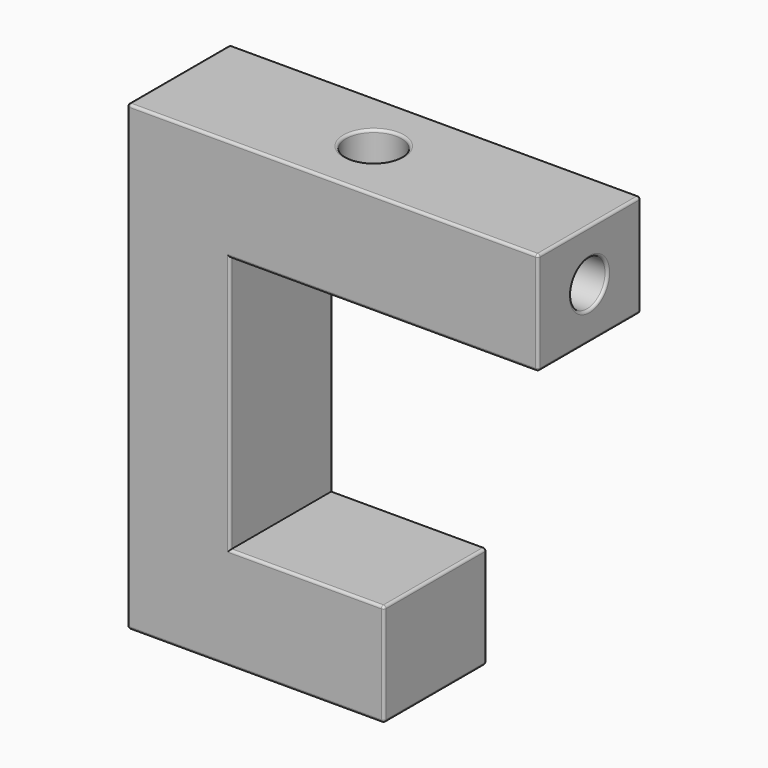
from build123d import *

# Parameters (mm, degrees)
F1_DEPTH = 25
F3_D     = 10.8
F3_DEPTH = 21
F3_TIP   = 3.2446473427
F5_D     = 8.8
F5_DEPTH = 21
F5_TIP   = 2.6437867237
F6_R     = 0.5


with BuildPart() as f1:
    # F0 (on Front) → F1 (new body)
    with BuildSketch(Plane.XZ):
        Polygon((0, -20), (0, 0), (-30, 0), (-30, 50), (30, 50), (30, 70), (-50, 70), (-50, -20), align=None)
    extrude(amount=F1_DEPTH)

    # F3 (one way)
    with BuildSketch(Plane(origin=(0, 0, 50), x_dir=(1, 0, 0), z_dir=(0, 0, -1))):
        with Locations((-12, 12.5)):
            Circle(F3_D / 2)
    extrude(amount=-F3_DEPTH, mode=Mode.SUBTRACT)
    with Locations(Plane(origin=(0, 0, 50), x_dir=(1, 0, 0), z_dir=(0, 0, -1))):
        with Locations((-12, 12.5)):
            with Locations((0, 0, -(F3_DEPTH + F3_TIP / 2))):  # 118° drill point
                Cone(0, F3_D / 2, F3_TIP, mode=Mode.SUBTRACT)

    # F5
    with Locations(Plane.YZ.offset(30)):
        with Locations((-12.5, 60)):
            Hole(F5_D / 2, depth=F5_DEPTH)
            with Locations((0, 0, -(F5_DEPTH + F5_TIP / 2))):  # 118° drill point
                Cone(0, F5_D / 2, F5_TIP, mode=Mode.SUBTRACT)

    # F6
    f6_edges = [f1.edges().sort_by_distance(p)[0] for p in [
        (0, -25, -10),
        (-15, -25, 0),
        (-30, -25, 25),
        (0, -25, 50),
        (30, -25, 60),
        (-10, -25, 70),
        (-50, -25, 25),
        (-25, -25, -20),
        (0, 0, -10),
        (-15, 0, 0),
        (-30, 0, 25),
        (0, 0, 50),
        (30, 0, 60),
        (-10, 0, 70),
        (-50, 0, 25),
        (-25, 0, -20),
        (30, -12.5, 70),
        (30, -12.5, 50),
        (0, -12.5, -20),
        (0, -12.5, 0),
        (-50, -12.5, -20),
        (-50, -12.5, 70),
        (-17.4, -12.5, 50),
        (30, -16.9, 60),
        (-17.4, -12.5, 70),
    ]]
    fillet(f6_edges, radius=F6_R)


solid = f1.part
